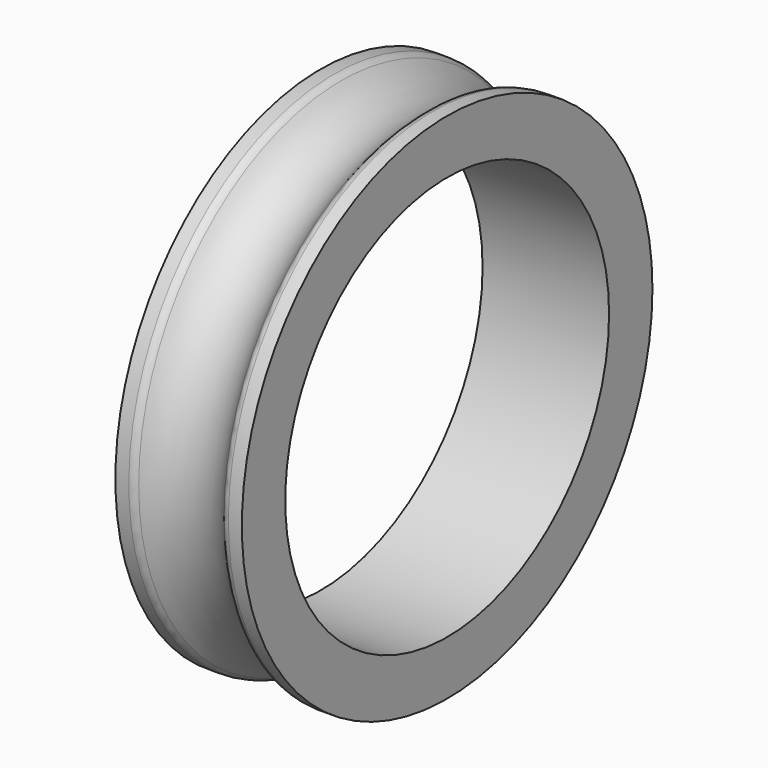
from build123d import *

# Parameters (mm, degrees)
F2_R = 0.5


with BuildPart() as f1:
    # F0 (on Top) → F1 (revolve)
    with BuildSketch(Plane.XY):
        with BuildLine():
            Line((-3.5, -1.5), (3.5, -1.5))
            Line((3.5, -1.5), (3.5, 1.5))
            Line((3.5, 1.5), (2.5, 1.5))
            ThreePointArc((2.5, 1.5), (0, 0.1583123952), (-2.5, 1.5))
            Line((-2.5, 1.5), (-3.5, 1.5))
            Line((-3.5, 1.5), (-3.5, -1.5))
        make_face()
    revolve(axis=Axis((0, -12.7, 0), (1, 0, 0)))

    # F2
    f2_edges = [f1.edges().sort_by_distance(p)[0] for p in [
        (-2.5, -26.9, 0),
        (2.5, -26.9, 0),
    ]]
    fillet(f2_edges, radius=F2_R)


solid = f1.part
